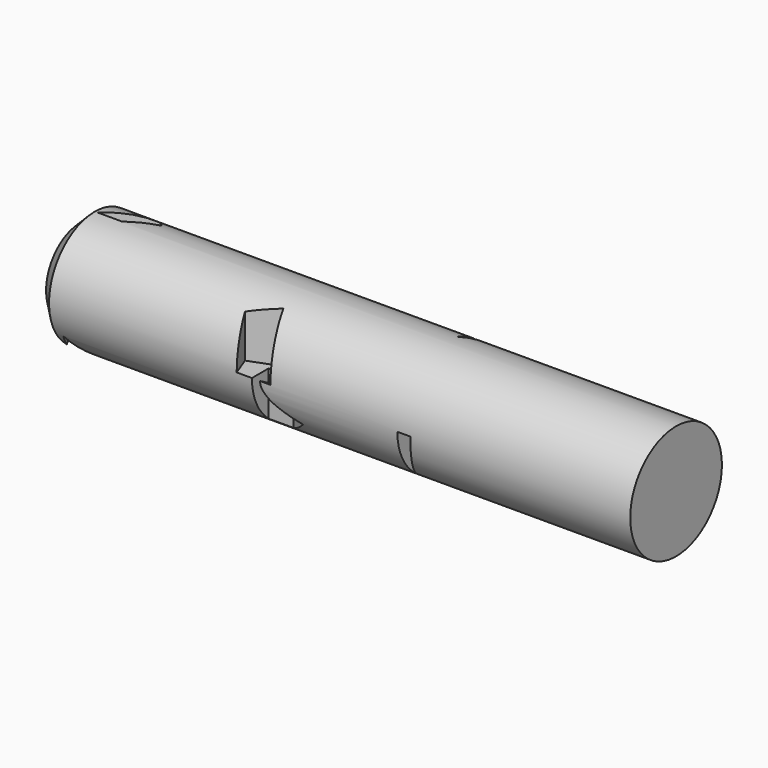
from build123d import *

# Parameters (mm, degrees)
F0_R        = 19.5387268204
F1_DEPTH    = 101.6
F3_DEPTH    = 38.1
F5_DEPTH    = 25.4
F7_DEPTH    = 25.4
F8_T2_ANGLE = 300.1049055837
F8_T4_ANGLE = 131.5703123603


# Not quite as in the source:
# - a fillet or chamfer that OpenCascade refuses, or shapes differently, is made with other operations: its cross-section is extruded or revolved along the edge and cut away or added


with BuildPart() as f1:
    # F0 (on Right) → F1 (new body, symmetric)
    with BuildSketch(Plane.YZ):
        Circle(F0_R)
    extrude(amount=F1_DEPTH, both=True)

    # F2 (on Top) → F3 (cut)
    with BuildSketch(Plane.XY):
        Polygon((-49.3527501822, 13.7382084504), (-37.9295572639, 12.1708353981), (-49.3527501822, 22.1678428352), align=None)
    extrude(amount=-F3_DEPTH, mode=Mode.SUBTRACT)

    # F4 (on Top) → F5 (cut)
    with BuildSketch(Plane.XY):
        Polygon((-103.1729057431, 0), (-93.9432457089, -16.6200213134), (-87.8715068102, -10.7566714287), align=None)
        Polygon((22.2135502845, -11.3549903035), (22.2135502845, -20.1754160225), (26.9660595804, -20.1754160225), align=None)
        Polygon((-77.9622271657, 12.2874397784), (-86.7114588618, 22.1413038671), (-82.0683091879, 6.1605265364), (-65.0239139795, 12.2874397784), (-72.4504972355, 17.1812968249), align=None)
        Polygon((0, 22.1413038671), (-8.541457355, 12.2874397784), (0, 12.2874397784), align=None)
        Polygon((-27.3653976619, -12.4159986153), (-27.3653976619, -20.1754160225), (-12.2119756415, -16.6692733765), (-18.8832655549, -12.4159986153), align=None)
    extrude(amount=-F5_DEPTH, mode=Mode.SUBTRACT)

    # F6 (on Top) → F7 (cut)
    with BuildSketch(Plane.XY):
        Polygon((-32.052900187, -20.8235712349), (-20.0643315911, -22.1631750464), (-25.0567086041, -9.0359868482), (-35.0853319095, -12.8499542954), align=None)
        Polygon((23.2855007052, 4.9763009883), (30.9053044766, 17.5455939025), (23.2855007052, 13.3292628452), align=None)
        Polygon((-78.8187682629, 6.2337135896), (-83.6249142885, 11.739499867), (-95.4798087478, 0), (-87.3620659113, 0), align=None)
        Polygon((-32.4846748263, 17.5455939025), (-37.5734344125, 11.739499867), (-27.39591524, 11.739499867), align=None)
    extrude(amount=F7_DEPTH, mode=Mode.SUBTRACT)

    # F8: chamfer of 5.08 on 1 edges, made by hand

    # F8_s1 → F8_t2 (revolve, cut)
    with BuildSketch(Plane.XY):
        Polygon((-96.52, 19.5387268204), (-101.6, 14.4587268204), (-101.6, 19.5387268204), align=None)
    revolve(axis=Axis((-101.6, 0, 0), (1, 0, 0)), revolution_arc=F8_T2_ANGLE, mode=Mode.SUBTRACT)

    # F8_s3 → F8_t4 (revolve, cut)
    with BuildSketch(Plane(origin=(0, 0, 0), x_dir=(1, 0, 0), z_dir=(0, -0.7481420015, 0.6635386542))):
        Polygon((-96.52, -19.5387268204), (-101.6, -14.4587268204), (-101.6, -19.5387268204), align=None)
    revolve(axis=Axis((-101.6, 0, 0), (1, 0, 0)), revolution_arc=F8_T4_ANGLE, mode=Mode.SUBTRACT)


solid = f1.part
